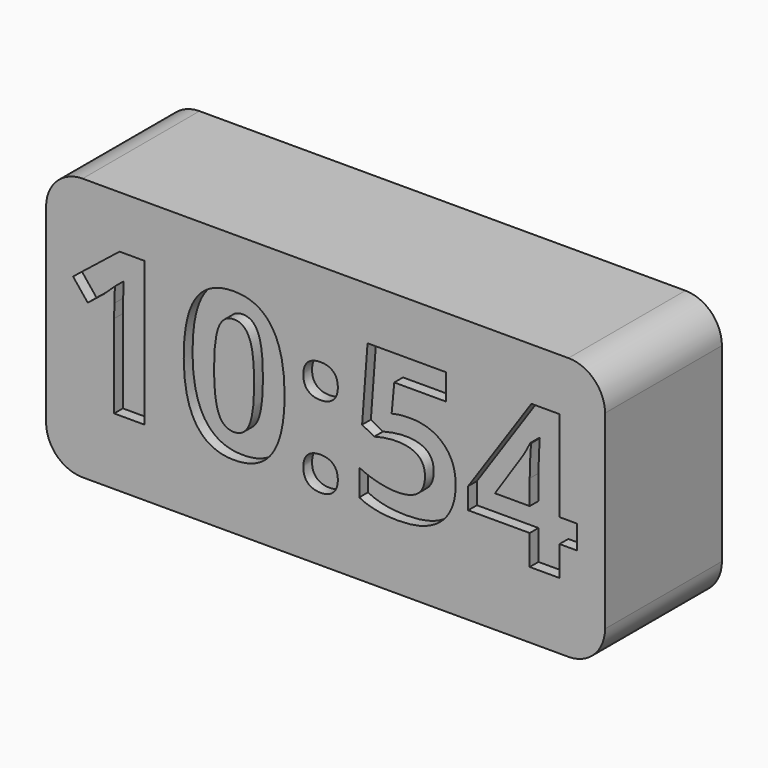
from build123d import *

# Parameters (mm, degrees)
F1_DEPTH     = 40
F2_TEXT_SIZE = 55.3065186573
F3_DEPTH     = 3


# Not quite as in the source:
# - Text() gives the source's letters only with a copy of the font that has no kerning and outlines rounded to 1/6400 em; it was checked with that copy


with BuildPart() as f1:
    # F0 (on Front) → F1 (new body)
    with BuildSketch(Plane.XZ):
        with BuildLine():
            Line((-66.5, -36), (66.5, -36))
            ThreePointArc((66.5, -36), (73.5710678119, -33.0710678119), (76.5, -26))
            Line((76.5, -26), (76.5, 26))
            ThreePointArc((76.5, 26), (73.5710678119, 33.0710678119), (66.5, 36))
            Line((66.5, 36), (-66.5, 36))
            ThreePointArc((-66.5, 36), (-73.5710678119, 33.0710678119), (-76.5, 26))
            Line((-76.5, 26), (-76.5, -26))
            ThreePointArc((-76.5, -26), (-73.5710678119, -33.0710678119), (-66.5, -36))
        make_face()
    extrude(amount=F1_DEPTH)

    # F2 (on face) → F3 (cut)
    with BuildSketch(Plane.XZ.offset(40)):
        with Locations((-72.3824062928, -17.7884902805)):
            Text('10:54', F2_TEXT_SIZE, font='Open Sans', font_style=FontStyle.BOLD, text_align=(TextAlign.LEFT, TextAlign.BOTTOM))
    extrude(amount=-F3_DEPTH, mode=Mode.SUBTRACT)


solid = f1.part
